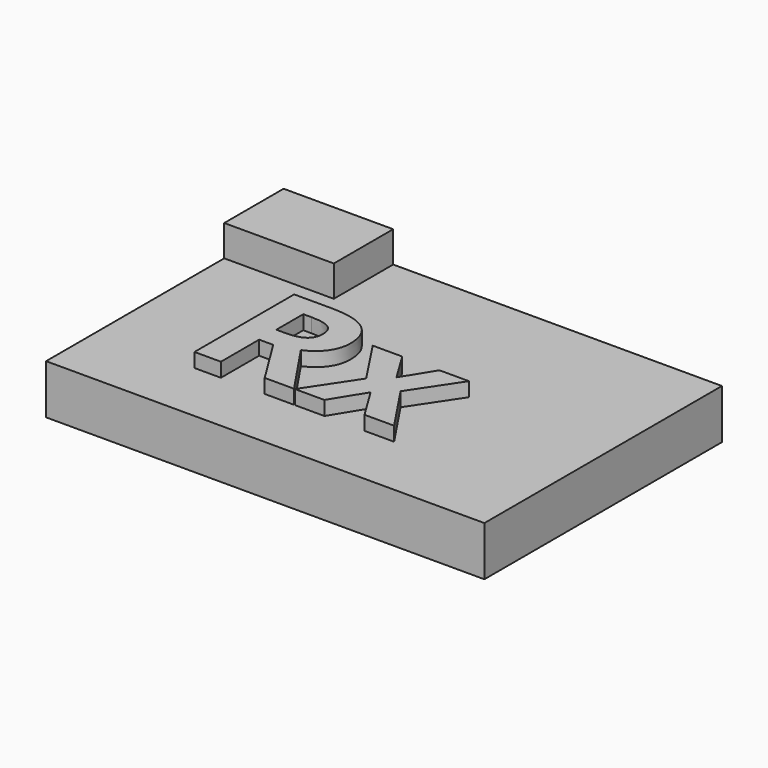
from build123d import *

# Parameters (mm, degrees)
F0_W         = 31
F0_H         = 21
F1_DEPTH     = 3.5
F2_W         = 7.75
F2_H         = 5.25
F3_DEPTH     = 2.2
F4_TEXT_SIZE = 12.3466837168
F5_DEPTH     = 1


# Not quite as in the source:
# - Text() gives the source's letters only with a copy of the font that has no kerning and outlines rounded to 1/6400 em; it was checked with that copy


with BuildPart() as f1:
    # F0 (on Top) → F1 (new body)
    with BuildSketch(Plane.XY):
        with Locations((13.0588222825, 10.5)):
            Rectangle(F0_W, F0_H)
    extrude(amount=F1_DEPTH)

    # F2 (on face) → F3 (join)
    with BuildSketch(Plane.XY.offset(3.5)):
        with Locations((1.4338222825, 18.375)):
            Rectangle(F2_W, F2_H)
    extrude(amount=F3_DEPTH)

    # F4 (on face) → F5 (join)
    with BuildSketch(Plane.XY.offset(3.5)):
        with Locations((3.3606998622, 4.479337018)):
            Text('Rx', F4_TEXT_SIZE, font='Open Sans', font_style=FontStyle.BOLD, text_align=(TextAlign.LEFT, TextAlign.BOTTOM))
    extrude(amount=F5_DEPTH)


solid = f1.part
